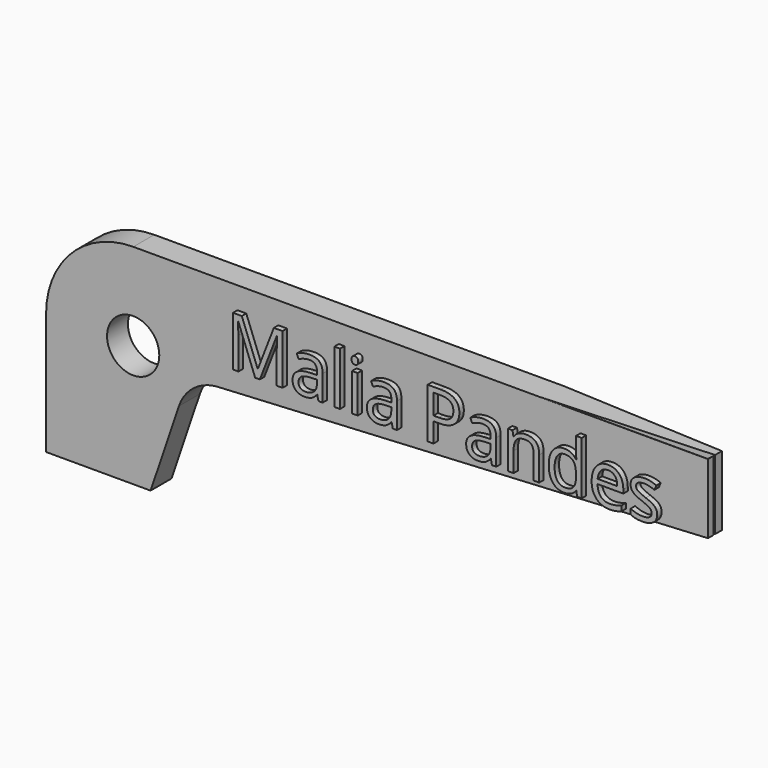
from build123d import *

# Parameters (mm, degrees)
F1_DEPTH     = 2.38125
F2_R         = 2.38125
F3_DEPTH     = 2.38225
F6_DEPTH     = 25.4
F7_TEXT_SIZE = 6.3789312653
F8_DEPTH     = 0.508


# Not quite as in the source:
# - Text() gives the source's letters only with a copy of the font that has no kerning and outlines rounded to 1/6400 em; it was checked with that copy


with BuildPart() as f1:
    # F0 (on Front) → F1 (new body)
    with BuildSketch(Plane.XZ):
        with BuildLine():
            Line((60.325, 19.05), (7.9502, 19.05))
            ThreePointArc((7.9502, 19.05), (2.3285596682, 16.7214403318), (0, 11.0998))
            Line((0, 11.0998), (0, 0))
            Line((0, 0), (9.525, 0))
            Line((9.525, 0), (12.1103451907, 7.6262422093))
            ThreePointArc((12.1103451907, 7.6262422093), (13.4737562991, 9.5178776332), (15.6634210502, 10.3194652484))
            Line((15.6634210502, 10.3194652484), (60.325, 12.7))
            Line((60.325, 12.7), (60.325, 19.05))
        make_face()
    extrude(amount=F1_DEPTH)

    # F2 (on face) → F3 (cut, through all)
    with BuildSketch(Plane.XZ.offset(2.38125)):
        with Locations((7.9375, 11.1125)):
            Circle(F2_R)
    extrude(amount=-F3_DEPTH, mode=Mode.SUBTRACT)

    # F5 (on face) → F6 (cut)
    with BuildSketch(Plane.XY.offset(19.05)):
        Polygon((60.3554546209, 0), (45.2742046209, 0), (60.3554546209, -0.79375), align=None)
        Polygon((60.3353911006, -1.5732463956), (45.0514033437, -2.3659453727), (60.2945573628, -2.3659453727), align=None)
    extrude(amount=-F6_DEPTH, mode=Mode.SUBTRACT)

    # F7 (on face) → F8 (join)
    with BuildSketch(Plane.XZ.offset(2.38125)):
        with Locations((16.8209241802, 12.4968581233)):
            Text('Malia Pandes', F7_TEXT_SIZE, font='Open Sans', text_align=(TextAlign.LEFT, TextAlign.BOTTOM))
    extrude(amount=F8_DEPTH)


solid = f1.part
